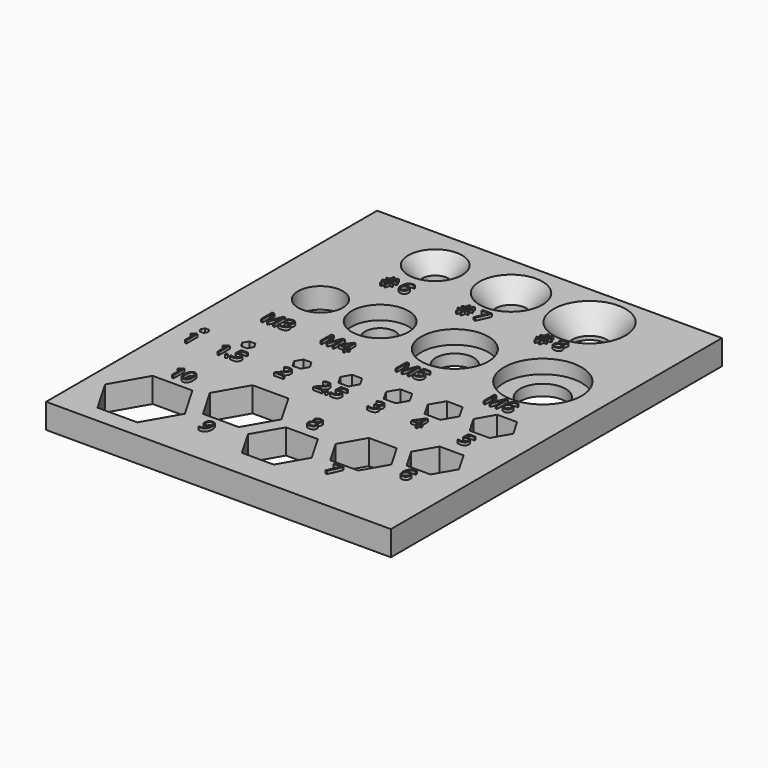
from build123d import *

# Parameters (mm, degrees)
F0_W           = 50
F0_H           = 60
F1_DEPTH       = 3.6
F2_D           = 3.3
F2_CBORE_D     = 6.5
F2_CBORE_DEPTH = 3
F3_D           = 5.5
F3_CBORE_D     = 9.75
F3_CBORE_DEPTH = 2
F4_D           = 4.4
F4_CBORE_D     = 8.25
F4_CBORE_DEPTH = 2
F5_D           = 6.6
F5_CBORE_D     = 11.25
F5_CBORE_DEPTH = 2
F6_D           = 3.7973
F6_CSINK_D     = 7.7978
F6_CSINK_ANGLE = 82
F7_D           = 4.4958
F7_CSINK_D     = 9.1186
F7_CSINK_ANGLE = 82
F8_D           = 5.1054
F8_CSINK_D     = 10.4394
F8_CSINK_ANGLE = 82
F9_TEXT_SIZE   = 2.7777777778
F10_DEPTH      = 0.4


# Not quite as in the source:
# - Text() gives the source's letters only with a copy of the font that has no kerning and outlines rounded to 1/6400 em; it was checked with that copy


with BuildPart() as f1:
    # F0 (on Top) → F1 (new body)
    with BuildSketch(Plane.XY):
        with Locations((-35.5663247406, 12.2679720819)):
            Rectangle(F0_W, F0_H)
        Polygon((-58.0040210032, -10.2288579755), (-55.1172696572, -5.2288579755), (-49.3437669653, -5.2288579755), (-46.4570156194, -10.2288579755), (-49.3437669653, -15.2288579755), (-55.1172696572, -15.2288579755), align=None, mode=Mode.SUBTRACT)
        Polygon((-47.4401509204, -4.4590865591), (-44.8420747091, 0.0409134409), (-39.6459222864, 0.0409134409), (-37.047846075, -4.4590865591), (-39.6459222864, -8.9590865591), (-44.8420747091, -8.9590865591), align=None, mode=Mode.SUBTRACT)
        Polygon((-58.0348792776, 7.0787493736), (-57.746204143, 7.5787493736), (-57.1688538738, 7.5787493736), (-56.8801787392, 7.0787493736), (-57.1688538738, 6.5787493736), (-57.746204143, 6.5787493736), align=None, mode=Mode.SUBTRACT)
        Polygon((-52.2727739966, 7.4539162517), (-51.8397612947, 8.2039162517), (-50.973735891, 8.2039162517), (-50.5407231891, 7.4539162517), (-50.973735891, 6.7039162517), (-51.8397612947, 6.7039162517), align=None, mode=Mode.SUBTRACT)
        Polygon((-44.8565355151, 7.5787493736), (-44.2791852459, 8.5787493736), (-43.1244847075, 8.5787493736), (-42.5471344383, 7.5787493736), (-43.1244847075, 6.5787493736), (-44.2791852459, 6.5787493736), align=None, mode=Mode.SUBTRACT)
        Polygon((-38.3565582594, 7.8287493736), (-37.6348704229, 9.0787493736), (-36.1914947499, 9.0787493736), (-35.4698069135, 7.8287493736), (-36.1914947499, 6.5787493736), (-37.6348704229, 6.5787493736), align=None, mode=Mode.SUBTRACT)
        Polygon((-37.7410026724, -9.6651211344), (-35.4316015956, -5.6651211344), (-30.8127994421, -5.6651211344), (-28.5033983653, -9.6651211344), (-30.8127994421, -13.6651211344), (-35.4316015956, -13.6651211344), align=None, mode=Mode.SUBTRACT)
        Polygon((-28.5007934253, -5.3333315384), (-26.4800674831, -1.8333315384), (-22.4386155988, -1.8333315384), (-20.4178896566, -5.3333315384), (-22.4386155988, -8.8333315384), (-26.4800674831, -8.8333315384), align=None, mode=Mode.SUBTRACT)
        Polygon((-32.0231759859, 8.2032496706), (-31.1571505821, 9.7032496706), (-29.4250997746, 9.7032496706), (-28.5590743708, 8.2032496706), (-29.4250997746, 6.7032496706), (-31.1571505821, 6.7032496706), align=None, mode=Mode.SUBTRACT)
        Polygon((-26.3890696895, 8.728862956), (-25.2153481962, 10.7177599341), (-22.906052141, 10.6957357931), (-21.7704775791, 8.6848146739), (-22.9441990723, 6.6959176958), (-25.2534951275, 6.7179418368), align=None, mode=Mode.SUBTRACT)
        Polygon((-20.6368796404, -1.4665466473), (-18.9048288328, 1.5334533527), (-15.4407272177, 1.5334533527), (-13.7086764101, -1.4665466473), (-15.4407272177, -4.4665466473), (-18.9048288328, -4.4665466473), align=None, mode=Mode.SUBTRACT)
        Polygon((-20.1344971132, 9.1959176958), (-18.6911214402, 11.6959176958), (-15.8043700943, 11.6959176958), (-14.3609944213, 9.1959176958), (-15.8043700943, 6.6959176958), (-18.6911214402, 6.6959176958), align=None, mode=Mode.SUBTRACT)
    extrude(amount=-F1_DEPTH)

    # F2 (through all)
    with Locations(Plane.XY):
        with Locations((-51.9835911691, 21.2722811848)):
            CounterBoreHole(F2_D / 2, F2_CBORE_D / 2, F2_CBORE_DEPTH)

    # F3 (through all)
    with Locations(Plane.XY):
        with Locations((-32.5039085001, 21.2722811848)):
            CounterBoreHole(F3_D / 2, F3_CBORE_D / 2, F3_CBORE_DEPTH)

    # F4 (through all)
    with Locations(Plane.XY):
        with Locations((-43.3324351907, 21.2722811848)):
            CounterBoreHole(F4_D / 2, F4_CBORE_D / 2, F4_CBORE_DEPTH)

    # F5 (through all)
    with Locations(Plane.XY):
        with Locations((-19.7411887348, 21.2722811848)):
            CounterBoreHole(F5_D / 2, F5_CBORE_D / 2, F5_CBORE_DEPTH)

    # F6 (through all)
    with Locations(Plane.XY):
        with Locations((-47.075338196, 35.9364151955)):
            CounterSinkHole(F6_D / 2, F6_CSINK_D / 2, counter_sink_angle=F6_CSINK_ANGLE)

    # F7 (through all)
    with Locations(Plane.XY):
        with Locations((-36.0843203962, 35.9364151955)):
            CounterSinkHole(F7_D / 2, F7_CSINK_D / 2, counter_sink_angle=F7_CSINK_ANGLE)

    # F8 (through all)
    with Locations(Plane.XY):
        with Locations((-24.6927775443, 35.9364151955)):
            CounterSinkHole(F8_D / 2, F8_CSINK_D / 2, counter_sink_angle=F8_CSINK_ANGLE)

    # F9 (on Top) → F10 (join)
    with BuildSketch(Plane.XY):
        with Locations((-54.0402317941, 12.7475582494)):
            Text('M3', F9_TEXT_SIZE, font='Open Sans', text_align=(TextAlign.LEFT, TextAlign.BOTTOM))
        with Locations((-45.4426782462, 12.7475582494)):
            Text('M4', F9_TEXT_SIZE, font='Open Sans', text_align=(TextAlign.LEFT, TextAlign.BOTTOM))
        with Locations((-34.5620682223, 12.7475582494)):
            Text('M5', F9_TEXT_SIZE, font='Open Sans', text_align=(TextAlign.LEFT, TextAlign.BOTTOM))
        with Locations((-21.8115012348, 12.7475582494)):
            Text('M6', F9_TEXT_SIZE, font='Open Sans', text_align=(TextAlign.LEFT, TextAlign.BOTTOM))
        with Locations((-49.1497739599, 28.1292927117)):
            Text('# 6', F9_TEXT_SIZE, font='Open Sans', text_align=(TextAlign.LEFT, TextAlign.BOTTOM))
        with Locations((-38.1559349795, 28.1292927117)):
            Text('# 7', F9_TEXT_SIZE, font='Open Sans', text_align=(TextAlign.LEFT, TextAlign.BOTTOM))
        with Locations((-26.7630900443, 28.1292927117)):
            Text('# 8', F9_TEXT_SIZE, font='Open Sans', text_align=(TextAlign.LEFT, TextAlign.BOTTOM))
        with Locations((-58.0323988001, 3.3823668467)):
            Text('1', F9_TEXT_SIZE, font='Open Sans', text_align=(TextAlign.LEFT, TextAlign.BOTTOM))
        with Locations((-53.3746305373, 3.3823668467)):
            Text('1.5', F9_TEXT_SIZE, font='Open Sans', text_align=(TextAlign.LEFT, TextAlign.BOTTOM))
        with Locations((-44.5115137961, 3.3823668467)):
            Text('2', F9_TEXT_SIZE, font='Open Sans', text_align=(TextAlign.LEFT, TextAlign.BOTTOM))
        with Locations((-38.8810645309, 3.3823668467)):
            Text('2.5', F9_TEXT_SIZE, font='Open Sans', text_align=(TextAlign.LEFT, TextAlign.BOTTOM))
        with Locations((-31.0938595533, 3.3823668467)):
            Text('3', F9_TEXT_SIZE, font='Open Sans', text_align=(TextAlign.LEFT, TextAlign.BOTTOM))
        with Locations((-24.9361104398, 3.3823668467)):
            Text('4', F9_TEXT_SIZE, font='Open Sans', text_align=(TextAlign.LEFT, TextAlign.BOTTOM))
        with Locations((-18.0519992395, 3.3823668467)):
            Text('5', F9_TEXT_SIZE, font='Open Sans', text_align=(TextAlign.LEFT, TextAlign.BOTTOM))
        with Locations((-17.9891842753, -7.3743375465)):
            Text('6', F9_TEXT_SIZE, font='Open Sans', text_align=(TextAlign.LEFT, TextAlign.BOTTOM))
        with Locations((-25.2729266104, -11.7057488747)):
            Text('7', F9_TEXT_SIZE, font='Open Sans', text_align=(TextAlign.LEFT, TextAlign.BOTTOM))
        with Locations((-33.934483505, -4.2360577714)):
            Text('8', F9_TEXT_SIZE, font='Open Sans', text_align=(TextAlign.LEFT, TextAlign.BOTTOM))
        with Locations((-43.0536773172, -12.3721194902)):
            Text('9', F9_TEXT_SIZE, font='Open Sans', text_align=(TextAlign.LEFT, TextAlign.BOTTOM))
        with Locations((-53.8396762974, -4.2155877668)):
            Text('10', F9_TEXT_SIZE, font='Open Sans', text_align=(TextAlign.LEFT, TextAlign.BOTTOM))
    extrude(amount=F10_DEPTH)


solid = f1.part
